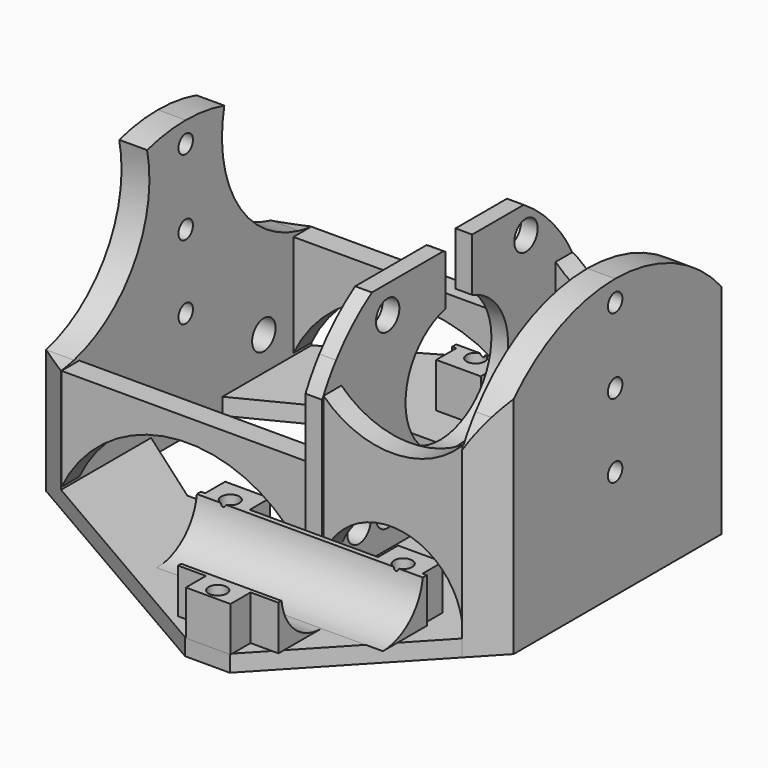
from build123d import *

# Parameters (mm, degrees)
F0_R       = 1.625
F1_DEPTH   = 8
F1_FACE1_W = 9.85
F1_FACE1_H = 8
F3_DEPTH   = 40.501
F5_W       = 3
F5_H       = 56.3
F6_DEPTH   = 3
F7_DEPTH   = 42
F8_R       = 1.625
F9_DEPTH   = 25
F10_R      = 2.625
F11_DEPTH  = 25
F13_DEPTH  = 47
F15_DEPTH  = 4
F16_START  = -52
F16_DEPTH  = 4
F17_R      = 1.625
F18_DEPTH  = 25
F19_START  = -21.2
F19_DEPTH  = 62.8
F21_DEPTH  = 25
F22_DEPTH  = 60.2


# Not quite as in the source:
# - a feature names something its author has since deleted; it is built from what else it names


with BuildPart() as f1:
    # F0 (on Top) → F1 (new body)
    with BuildSketch(Plane.XY):
        Polygon((11.5, 23.65), (19.5, 23.65), (19.5, 28.15), (20.25, 28.15), (20.25, 38), (9.25, 38), (9.25, 47.65), (4.25, 47.65), (4.25, 52.15), (-3.75, 52.15), (-3.75, 47.65), (-8.75, 47.65), (-8.75, 38), (-20.25, 38), (-20.25, 28.15), (-19.5, 28.15), (-19.5, 23.65), (-11.5, 23.65), (-11.5, 28.15), (11.5, 28.15), align=None)
        with Locations((-15.5, 27.4999994636)):
            Circle(F0_R, mode=Mode.SUBTRACT)
        with Locations((15.5, 27.4999994636)):
            Circle(F0_R, mode=Mode.SUBTRACT)
        with Locations((0.25, 49.9999994636)):
            Circle(F0_R, mode=Mode.SUBTRACT)
    extrude(amount=F1_DEPTH)

    # F2 (on face) + F1_face1 (on face) → F3 (cut, through all)
    with BuildSketch(Plane.YZ.offset(20.25)):
        with BuildLine():
            Line((38, 8), (38, 0))
            ThreePointArc((38, 0), (44.9534101129, 3.2859744661), (46.8293250961, 10.744424933))
            Line((46.8293250961, 10.744424933), (29.1706749039, 10.744424933))
            ThreePointArc((29.1706749039, 10.744424933), (29.0078837481, 9.376623569), (29.05572809, 8))
            Line((29.05572809, 8), (38, 8))
        make_face()
        with BuildLine():
            ThreePointArc((29.05572809, 8), (32, 2.2917960675), (38, 0))
            Line((38, 0), (38, 8))
            Line((38, 8), (29.05572809, 8))
        make_face()
    with BuildSketch(Plane(origin=(-20.25, 33.075, 4), x_dir=(0, -1, 0), z_dir=(-1, 0, 0))):
        Rectangle(F1_FACE1_W, F1_FACE1_H)
    extrude(amount=-F3_DEPTH, dir=(1, 0, 0), mode=Mode.SUBTRACT)


with BuildPart() as f4_1:
    # F4: instance of F1
    add(f1.part.mirror(Plane.XZ))


with BuildPart() as f6:
    # F5 (on Top) → F6 (new body)
    with BuildSketch(Plane.XY):
        Polygon((4, 52), (-4, 52), (-45.5, 28.1937253379), (-45.5, 8.2134563482), (-29.9130736956, 16.1451932328), (-4.5, 16.159927385), (-4.5, -18.252106842), (-30.5883444961, -18.267232507), (-45.5, -7.7602324311), (-45.5, -27.9429632097), (-4, -52), (4, -52), (26.5, -28.0708628145), (26.5, 28.963479296), align=None)
        Rectangle(F5_W, F5_H, mode=Mode.SUBTRACT)
        Rectangle(F5_W, F5_H)
        Polygon((31.5, 23.8442524728), (26.5, 28.963479296), (26.5, -28.0708628145), (31.5, -22.7532767733), align=None)
        Polygon((-45.5, 8.2134563482), (-45.5, 28.1937253379), (-50.5, 25.325499475), (-50.5, -25.0445250422), (-45.5, -27.9429632097), (-45.5, -7.7602324311), align=None)
    extrude(amount=-F6_DEPTH)

    # F0 (on Top) + F8 (on face) → F9 (cut)
    with BuildSketch(Plane.XY):
        with Locations((-15.5, 27.4999994636)):
            Circle(F0_R)
        with Locations((0.25, 49.9999994636)):
            Circle(F0_R)
        with Locations((15.5, 27.4999994636)):
            Circle(F0_R)
    with BuildSketch(Plane.XY):
        with Locations((-15.5, -27.4999994636)):
            Circle(F8_R)
        with Locations((15.5, -27.4999994636)):
            Circle(F8_R)
        with Locations((0.25, -49.9999994636)):
            Circle(F8_R)
    extrude(amount=-F9_DEPTH, mode=Mode.SUBTRACT)


with BuildPart() as f7:
    # F5 (on Top) → F7 (new body)
    with BuildSketch(Plane.XY):
        Rectangle(F5_W, F5_H)
    extrude(amount=F7_DEPTH)

    # F10 (on face) → F11 (cut)
    with BuildSketch(Plane(origin=(-1.5, 0, 0), x_dir=(0, -1, 0), z_dir=(-1, 0, 0))):
        with Locations((-17.5160421579, 37)):
            Circle(F10_R)
        with Locations((13.4839578421, 37)):
            Circle(F10_R)
        with Locations((13.4839578421, 6)):
            Circle(F10_R)
        with Locations((-17.5160421579, 6)):
            Circle(F10_R)
        with BuildLine():
            ThreePointArc((-5.47296277, 32.4681219852), (-8.8166087873, 12.2262578471), (9.4839578421, 21.5))
            ThreePointArc((9.4839578421, 21.5), (6.9699306041, 28.6765098425), (0.52703723, 32.7152907776))
            ThreePointArc((0.52703723, 32.7152907776), (-2.4893808831, 32.990254586), (-5.47296277, 32.4681219852))
        make_face()
        with Locations((19.9137547576, 6.1115942442)):
            Circle(F10_R)
        with BuildLine():
            ThreePointArc((-5.47296277, 32.4681219852), (-2.4893808831, 32.990254586), (0.52703723, 32.7152907776))
            Line((0.52703723, 32.7152907776), (0.52703723, 42))
            Line((0.52703723, 42), (-5.47296277, 42))
            Line((-5.47296277, 42), (-5.47296277, 32.4681219852))
        make_face()
    extrude(amount=-F11_DEPTH, mode=Mode.SUBTRACT)


with BuildPart() as f1_1:
    add(f1.part)

    # F12: union F4_1, F6, F7
    add(f4_1.part)
    add(f6.part)
    add(f7.part)

    # F5 (on Top) → F13 (join)
    with BuildSketch(Plane.XY):
        Polygon((31.5, 23.8442524728), (26.5, 28.963479296), (26.5, -28.0708628145), (31.5, -22.7532767733), align=None)
        Polygon((-45.5, 8.2134563482), (-45.5, 28.1937253379), (-50.5, 25.325499475), (-50.5, -25.0445250422), (-45.5, -27.9429632097), (-45.5, -7.7602324311), align=None)
    extrude(amount=F13_DEPTH)

    # F14 (on face) → F15 (join)
    with BuildSketch(Plane(origin=(0, 28.15, 0), x_dir=(-1, 0, 0), z_dir=(0, 1, 0))):
        with BuildLine():
            ThreePointArc((-26.5, 1.0051795379), (-15.634804546, 13.2493790833), (-1.5, 4.9922491216))
            Line((-1.5, 4.9922491216), (-1.5, 8))
            Line((-1.5, 8), (-1.5, 18.7461301684))
            Line((-1.5, 18.7461301684), (-26.5, 18.7461301684))
            Line((-26.5, 18.7461301684), (-26.5, 1.0051795379))
        make_face()
        with BuildLine():
            Line((-26.5, 0), (-26.5, 1.0051795379))
            ThreePointArc((-26.5, 1.0051795379), (-26.5097882976, 0.502589769), (-26.5, 0))
        make_face()
        with BuildLine():
            Line((1.5, 18.7461301684), (1.5, 8))
            Line((1.5, 8), (1.5, 2.8133653057))
            ThreePointArc((1.5, 2.8133653057), (24.2130918491, 14.7122626951), (45.5, 0.4176538582))
            Line((45.5, 0.4176538582), (45.5, 18.7461301684))
            Line((45.5, 18.7461301684), (1.5, 18.7461301684))
        make_face()
        with BuildLine():
            Line((-26.5, 30.4596769747), (-26.5, 18.7461301684))
            Line((-26.5, 18.7461301684), (-1.5, 18.7461301684))
            Line((-1.5, 18.7461301684), (-1.5, 30.0831180066))
            ThreePointArc((-1.5, 30.0831180066), (-14.0789057826, 25.0327901758), (-26.5, 30.4596769747))
        make_face()
    extrude(amount=-F15_DEPTH)

    # F14 (on face) → F16 (join)
    with BuildSketch(Plane(origin=(0, 28.15, 0), x_dir=(-1, 0, 0), z_dir=(0, 1, 0)).offset(F16_START)):
        with BuildLine():
            ThreePointArc((-26.5, 1.0051795379), (-15.634804546, 13.2493790833), (-1.5, 4.9922491216))
            Line((-1.5, 4.9922491216), (-1.5, 8))
            Line((-1.5, 8), (-1.5, 18.7461301684))
            Line((-1.5, 18.7461301684), (-26.5, 18.7461301684))
            Line((-26.5, 18.7461301684), (-26.5, 1.0051795379))
        make_face()
        with BuildLine():
            Line((1.5, 18.7461301684), (1.5, 8))
            Line((1.5, 8), (1.5, 2.8133653057))
            ThreePointArc((1.5, 2.8133653057), (24.2130918491, 14.7122626951), (45.5, 0.4176538582))
            Line((45.5, 0.4176538582), (45.5, 18.7461301684))
            Line((45.5, 18.7461301684), (1.5, 18.7461301684))
        make_face()
        with BuildLine():
            Line((-26.5, 30.4596769747), (-26.5, 18.7461301684))
            Line((-26.5, 18.7461301684), (-1.5, 18.7461301684))
            Line((-1.5, 18.7461301684), (-1.5, 30.0831180066))
            ThreePointArc((-1.5, 30.0831180066), (-14.0789057826, 25.0327901758), (-26.5, 30.4596769747))
        make_face()
    extrude(amount=-F16_DEPTH)

    # F17 (on face) → F18 (cut)
    with BuildSketch(Plane(origin=(-50.5, 0, 0), x_dir=(0, -1, 0), z_dir=(-1, 0, 0))):
        with BuildLine():
            Line((-25.325499475, 47), (-25.325499475, 34.200413835))
            ThreePointArc((-25.325499475, 34.200413835), (-14.1881141246, 43.6183212915), (0, 47))
            Line((0, 47), (-25.325499475, 47))
        make_face()
        with BuildLine():
            Line((25.0445250422, 47), (0, 47))
            ThreePointArc((0, 47), (13.9784205751, 43.7233215332), (25.0445250422, 34.5759615057))
            Line((25.0445250422, 34.5759615057), (25.0445250422, 47))
        make_face()
        with Locations((0, 43.25)):
            Circle(F17_R)
        with Locations((0, 29.75)):
            Circle(F17_R)
        with Locations((0, 16.5)):
            Circle(F17_R)
        with BuildLine():
            Line((-30, 49.8921192791), (-30, 25))
            ThreePointArc((-30, 25), (-28.0426394393, 29.7932193887), (-25.325499475, 34.200413835))
            Line((-25.325499475, 34.200413835), (-25.325499475, 47))
            Line((-25.325499475, 47), (0, 47))
            Line((0, 47), (25.0445250422, 47))
            Line((25.0445250422, 47), (25.0445250422, 34.5759615057))
            ThreePointArc((25.0445250422, 34.5759615057), (27.935634841, 30.0018972539), (30, 25))
            Line((30, 25), (30, 50.0645951358))
            Line((30, 50.0645951358), (-30, 49.8921192791))
        make_face()
    extrude(amount=-F18_DEPTH, mode=Mode.SUBTRACT)

    # F17 (on face) → F19 (cut)
    with BuildSketch(Plane(origin=(-50.5, 0, 0), x_dir=(0, -1, 0), z_dir=(-1, 0, 0)).offset(F19_START)):
        with BuildLine():
            Line((-30, 49.8921192791), (-30, 25))
            ThreePointArc((-30, 25), (-28.0426394393, 29.7932193887), (-25.325499475, 34.200413835))
            Line((-25.325499475, 34.200413835), (-25.325499475, 47))
            Line((-25.325499475, 47), (-4.65e-08, 47))
            Line((-4.65e-08, 47), (25.0445250422, 47))
            Line((25.0445250422, 47), (25.0445250422, 34.5759615057))
            ThreePointArc((25.0445250422, 34.5759615057), (27.935634841, 30.0018972539), (30, 25))
            Line((30, 25), (30, 50.0645951358))
            Line((30, 50.0645951358), (-30, 49.8921192791))
        make_face()
        with Locations((0, 43.25)):
            Circle(F17_R)
        with Locations((0, 29.75)):
            Circle(F17_R)
        with Locations((0, 16.5)):
            Circle(F17_R)
        with BuildLine():
            Line((25.0445250422, 47), (-4.65e-08, 47))
            ThreePointArc((-4.65e-08, 47), (13.9784205543, 43.7233215435), (25.0445250422, 34.5759615057))
            Line((25.0445250422, 34.5759615057), (25.0445250422, 47))
        make_face()
        with BuildLine():
            Line((-25.325499475, 47), (-25.325499475, 34.200413835))
            ThreePointArc((-25.325499475, 34.200413835), (-14.1881141454, 43.618321281), (-4.65e-08, 47))
            Line((-4.65e-08, 47), (-25.325499475, 47))
        make_face()
    extrude(amount=-F19_DEPTH, mode=Mode.SUBTRACT)

    # F20 (on face) → F21 (cut)
    with BuildSketch(Plane(origin=(-50.5, 0, 0), x_dir=(0, -1, 0), z_dir=(-1, 0, 0))):
        with BuildLine():
            Line((-30.3553968664, 47.8501823954), (-30.4436534643, 18.6318717897))
            ThreePointArc((-30.4436534643, 18.6318717897), (-27.8671376383, 18.7854294921), (-25.325499475, 19.2349728339))
            Line((-25.325499475, 19.2349728339), (-25.325499475, 34.200413835))
            ThreePointArc((-25.325499475, 34.200413835), (-17.9491568504, 41.3759829588), (-8.6516256383, 45.7867806335))
            ThreePointArc((-8.6516256383, 45.7867806335), (-8.9061906115, 46.8251613964), (-9.2101147561, 47.8501823954))
            Line((-9.2101147561, 47.8501823954), (-30.3553968664, 47.8501823954))
        make_face()
        with BuildLine():
            Line((-25.325499475, 34.200413835), (-25.325499475, 19.2349728339))
            ThreePointArc((-25.325499475, 19.2349728339), (-11.5528931008, 29.0974117294), (-8.6516256383, 45.7867806335))
            ThreePointArc((-8.6516256383, 45.7867806335), (-17.9491568504, 41.3759829588), (-25.325499475, 34.200413835))
        make_face()
        with BuildLine():
            Line((30.4436534643, 47.8501823954), (9.2101147561, 47.8501823954))
            ThreePointArc((9.2101147561, 47.8501823954), (8.9061906115, 46.8251613964), (8.6516256383, 45.7867806335))
            ThreePointArc((8.6516256383, 45.7867806335), (17.7560766796, 41.5090862387), (25.0445250422, 34.5759615057))
            Line((25.0445250422, 34.5759615057), (25.0445250422, 19.3035224838))
            ThreePointArc((25.0445250422, 19.3035224838), (27.7235781794, 18.8028169058), (30.4436534643, 18.6318717897))
            Line((30.4436534643, 18.6318717897), (30.4436534643, 47.8501823954))
        make_face()
        with BuildLine():
            ThreePointArc((25.0445250422, 34.5759615057), (17.7560766796, 41.5090862387), (8.6516256383, 45.7867806335))
            ThreePointArc((8.6516256383, 45.7867806335), (11.4763854122, 29.220123644), (25.0445250422, 19.3035224838))
            Line((25.0445250422, 19.3035224838), (25.0445250422, 34.5759615057))
        make_face()
    extrude(amount=-F21_DEPTH, mode=Mode.SUBTRACT)

    # F10 (on face) → F22 (cut)
    with BuildSketch(Plane(origin=(-1.5, 0, 0), x_dir=(0, -1, 0), z_dir=(-1, 0, 0))):
        with Locations((13.4839578421, 6)):
            Circle(F10_R)
        with Locations((-17.5160421579, 6)):
            Circle(F10_R)
    extrude(amount=F22_DEPTH, mode=Mode.SUBTRACT)


solid = f1_1.part
